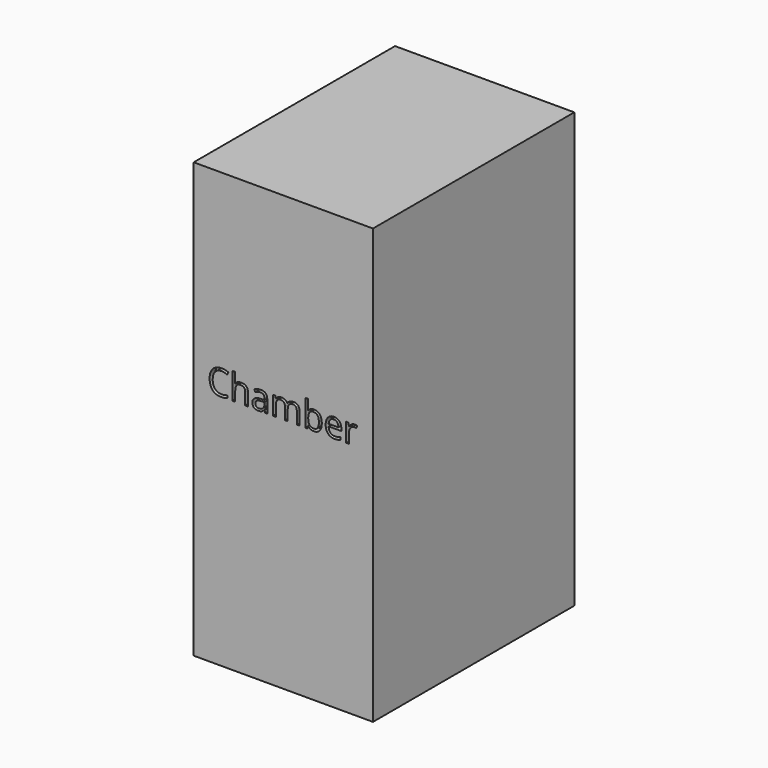
from build123d import *

# Parameters (mm, degrees)
F0_W         = 660.4
F0_H         = 927.1
F1_DEPTH     = 1600.2
F2_TEXT_SIZE = 128.0549985677
F3_DEPTH     = 25.4


# Not quite as in the source:
# - Text() gives the source's letters only with a copy of the font that has no kerning and outlines rounded to 1/6400 em; it was checked with that copy


with BuildPart() as f1:
    # F0 (on Top) → F1 (new body)
    with BuildSketch(Plane.XY):
        Rectangle(F0_W, F0_H)
    extrude(amount=F1_DEPTH)

    # F2 (on face) → F3 (cut)
    with BuildSketch(Plane.XZ.offset(463.55)):
        with Locations((-279.4, 873.0004010312)):
            Text('Chamber', F2_TEXT_SIZE, font='Open Sans', text_align=(TextAlign.LEFT, TextAlign.BOTTOM))
    extrude(amount=-F3_DEPTH, mode=Mode.SUBTRACT)


solid = f1.part
